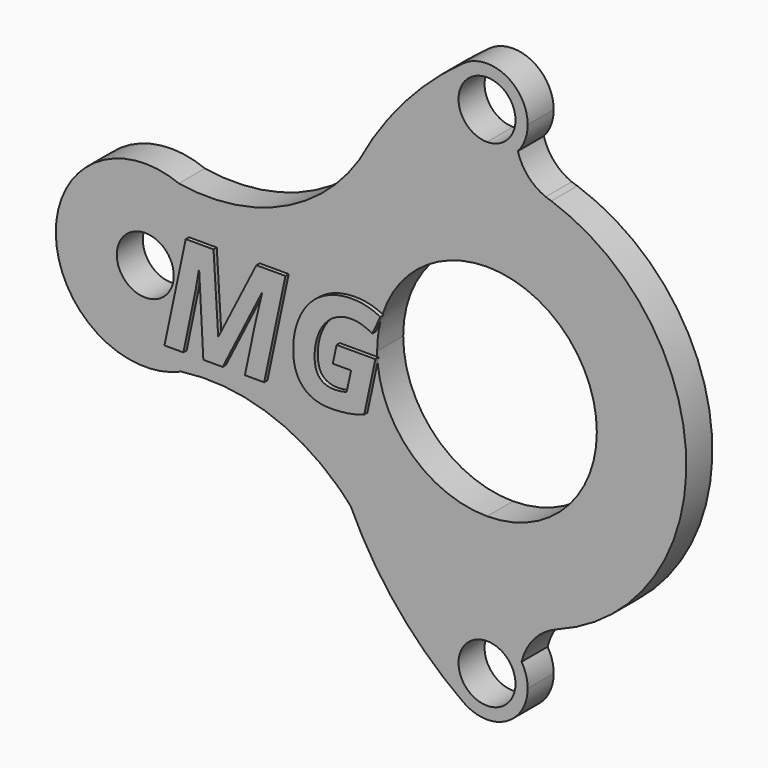
from build123d import *

# Parameters (mm, degrees)
F0_R         = 7
F1_DEPTH     = 8
F2_TEXT_SIZE = 34.6223047624
F3_DEPTH     = 1


# Not quite as in the source:
# - Text() gives the source's letters only with a copy of the font that has no kerning and outlines rounded to 1/6400 em; it was checked with that copy


with BuildPart() as f1:
    # F0 (on Front) → F1 (new body)
    with BuildSketch(Plane.XZ):
        with BuildLine():
            ThreePointArc((-27, 0), (-19.091883092, 19.091883092), (0, 27))
            Line((0, 27), (0, 51))
            ThreePointArc((0, 51), (-9.5219045714, 57.9449495367), (-5.8179797945, 69.1333333333))
            ThreePointArc((-5.8179797945, 69.1333333333), (-20.3036885116, 56.0077092026), (-31.4077984883, 39.9199341083))
            ThreePointArc((-31.4077984883, 39.9199341083), (-50.6722866613, 23.5474222274), (-75.7572943033, 20.3974950128))
            ThreePointArc((-75.7572943033, 20.3974950128), (-105.9974133255, -0.3373529122), (-75.1356847217, -20.135141287))
            ThreePointArc((-75.1356847217, -20.135141287), (-54.6476634602, -21.8938970781), (-36.8858160396, -32.2557990924))
            ThreePointArc((-36.8858160396, -32.2557990924), (-35.1260619993, -33.9815823016), (-33.4594951415, -35.7975164624))
            ThreePointArc((-33.4594951415, -35.7975164624), (-21.797298439, -54.2552684297), (-5.8179797945, -69.1333333333))
            ThreePointArc((-5.8179797945, -69.1333333333), (-9.5219045714, -57.9449495367), (0, -51))
            Line((0, -51), (0, -27))
            ThreePointArc((0, -27), (-19.091883092, -19.091883092), (-27, 0))
        make_face()
        with Locations((-84, 0)):
            Circle(F0_R, mode=Mode.SUBTRACT)
        with BuildLine():
            ThreePointArc((0, 27), (19.091883092, 19.091883092), (27, 0))
            ThreePointArc((27, 0), (19.091883092, -19.091883092), (0, -27))
            Line((0, -27), (0, -51))
            ThreePointArc((0, -51), (4.8652210438, -52.2633173232), (8.5011784824, -55.7340751609))
            ThreePointArc((8.5011784824, -55.7340751609), (11.5943334425, -49.7712467911), (17.0981072712, -45.9200906765))
            ThreePointArc((17.0981072712, -45.9200906765), (48.9953871337, 0.6723389193), (15.8316300135, 46.3719688078))
            ThreePointArc((15.8316300135, 46.3719688078), (15.1233786468, 46.5770456622), (14.4297488122, 46.8271539731))
            ThreePointArc((14.4297488122, 46.8271539731), (10.1049904693, 49.8497645431), (7.5884700978, 54.4873107264))
            ThreePointArc((7.5884700978, 54.4873107264), (4.1757099554, 51.9135570013), (0, 51))
            Line((0, 51), (0, 27))
        make_face()
        with BuildLine():
            ThreePointArc((8.5011784824, -55.7340751609), (4.8652210438, -52.2633173232), (0, -51))
            ThreePointArc((0, -51), (-9.5219045714, -57.9449495367), (-5.8179797945, -69.1333333333))
            ThreePointArc((-5.8179797945, -69.1333333333), (4.5727563928, -69.8932501917), (10, -61))
            ThreePointArc((10, -61), (9.6179983579, -58.2624632262), (8.5011784824, -55.7340751609))
        make_face()
        with BuildLine():
            ThreePointArc((7, -61), (-4.9497474683, -65.9497474683), (0, -54))
            ThreePointArc((0, -54), (4.9497474683, -56.0502525317), (7, -61))
        make_face(mode=Mode.SUBTRACT)
        with BuildLine():
            ThreePointArc((-5.8179797945, 69.1333333333), (-9.5219045714, 57.9449495367), (0, 51))
            ThreePointArc((0, 51), (4.1757099554, 51.9135570013), (7.5884700978, 54.4873107264))
            ThreePointArc((7.5884700978, 54.4873107264), (9.377758287, 57.5275873645), (10, 61))
            ThreePointArc((10, 61), (4.5727563928, 69.8932501917), (-5.8179797945, 69.1333333333))
        make_face()
        with BuildLine():
            ThreePointArc((7, 61), (4.9497474683, 56.0502525317), (0, 54))
            ThreePointArc((0, 54), (-4.9497474683, 65.9497474683), (7, 61))
        make_face(mode=Mode.SUBTRACT)
    extrude(amount=F1_DEPTH)

    # F2 (on face) → F3 (join)
    with BuildSketch(Plane.XZ.offset(8)):
        with Locations((-79.3781504035, -15.1551259914)):
            Text('MG', F2_TEXT_SIZE, font='Open Sans', font_style=FontStyle.BOLDITALIC, text_align=(TextAlign.LEFT, TextAlign.BOTTOM))
    extrude(amount=F3_DEPTH)


solid = f1.part
